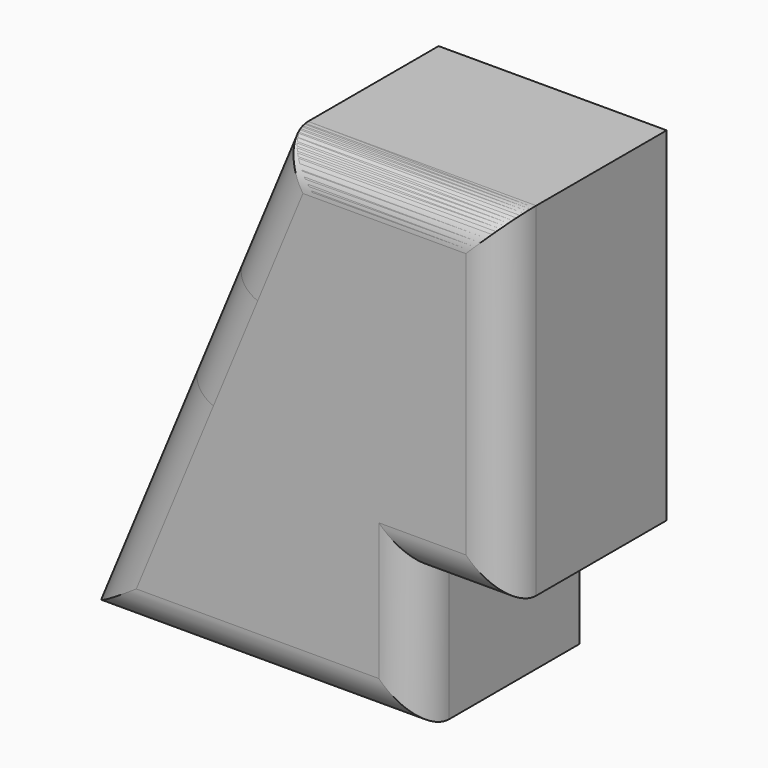
from build123d import *

# Parameters (mm, degrees)
F1_DEPTH = 25.4
F2_DEPTH = 25.4
F3_R     = 4.9056819587
F3_2_R   = 4.9056819587
F3_3_R   = 4.9056819587


with BuildPart() as f1:
    # F0 (on Front) → F1 (new body)
    with BuildSketch(Plane.XZ):
        Polygon((0, 26.3652000576), (6.7747447512, 26.3652000576), (28.6512039602, 26.3652000576), (28.6512039602, 43.1291982532), (0, 43.1291982532), (0, 34.7471991554), align=None)
    extrude(amount=F1_DEPTH)

    # F3
    f3_edges = [f1.edges().sort_by_distance(p)[0] for p in [
        (14.325602, -25.4, 26.3652),
        (28.651204, -25.4, 34.747199),
        (0, -25.4, 34.747199),
        (14.325602, -25.4, 43.129198),
    ]]
    fillet(f3_edges, radius=F3_R)


with BuildPart() as f1b:
    # F0 (on Front) → F1, piece 2 (new body)
    with BuildSketch(Plane.XZ):
        with BuildLine():
            ThreePointArc((16.3608330212, 0), (16.0455644423, 3.1963602544), (15.1119089765, 6.2695346107))
            ThreePointArc((15.1119089765, 6.2695346107), (-16.0455644423, -3.1963602544), (16.3608330212, 0))
        make_face()
    extrude(amount=F1_DEPTH)

    # F3#2
    f3_2_edges = [f1b.edges().sort_by_distance(p)[0] for p in [
        (-16.360833, -25.4, 0),
    ]]
    fillet(f3_2_edges, radius=F3_2_R)


with BuildPart() as f2:
    # F0 (on Front) → F2 (new body)
    with BuildSketch(Plane.XZ):
        Polygon((0, 26.3652000576), (6.7747447512, 26.3652000576), (28.6512039602, 26.3652000576), (28.6512039602, 43.1291982532), (0, 43.1291982532), (0, 34.7471991554), align=None)
        Polygon((0, 43.1291982532), (-6.9426662852, 26.3652000576), (0, 26.3652000576), (0, 34.7471991554), align=None)
        Polygon((-6.9426662852, 26.3652000576), (-12.4968001619, 12.9539994523), (6.7747447512, 26.3652000576), (0, 26.3652000576), align=None)
        Polygon((15.1119089765, 6.2695346107), (17.7129743557, 0), (28.6512039602, 26.3652000576), (6.7747447512, 26.3652000576), align=None)
        Polygon((28.6512039602, 26.3652000576), (17.7129743557, 0), (28.6512039602, 0), align=None)
        Polygon((-12.4968001619, 12.9539994523), (-24.9936003238, -17.2211993486), (17.7129743557, -17.2211993486), (17.7129743557, 0), (15.1119089765, 6.2695346107), (6.7747447512, 26.3652000576), align=None)
        with BuildLine():
            ThreePointArc((16.3608330212, 0), (-16.0455644423, -3.1963602544), (15.1119089765, 6.2695346107))
            ThreePointArc((15.1119089765, 6.2695346107), (16.0455644423, 3.1963602544), (16.3608330212, 0))
        make_face(mode=Mode.SUBTRACT)
        with BuildLine():
            ThreePointArc((16.3608330212, 0), (16.0455644423, 3.1963602544), (15.1119089765, 6.2695346107))
            ThreePointArc((15.1119089765, 6.2695346107), (-16.0455644423, -3.1963602544), (16.3608330212, 0))
        make_face()
    extrude(amount=F2_DEPTH)

    # F3#3
    f3_3_edges = [f2.edges().sort_by_distance(p)[0] for p in [
        (14.325602, -25.4, 43.129198),
        (-12.4968, -25.4, 12.953999),
        (-3.640313, -25.4, -17.221199),
        (17.712974, -25.4, -8.6106),
        (23.182089, -25.4, 0),
        (28.651204, -25.4, 21.564599),
    ]]
    fillet(f3_3_edges, radius=F3_3_R)


solid = Compound([f1.part, f1b.part, f2.part])
